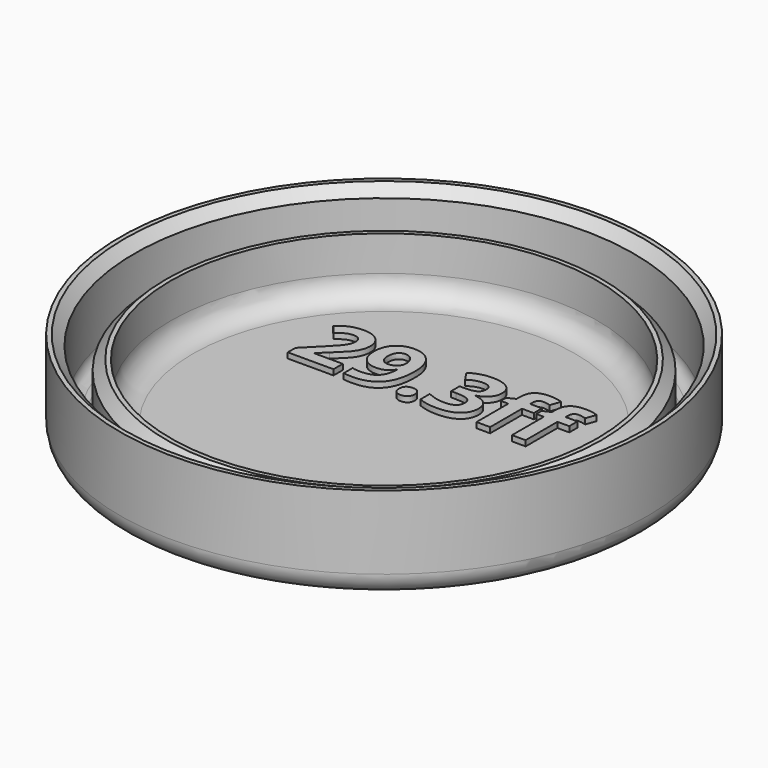
from build123d import *

# Parameters (mm, degrees)
F2_TEXT_SIZE = 8.3333333333
F3_DEPTH     = 0.5


# Not quite as in the source:
# - Text() gives the source's letters only with a copy of the font that has no kerning and outlines rounded to 1/6400 em; it was checked with that copy


with BuildPart() as f1:
    # F0 (on Front) → F1 (revolve)
    with BuildSketch(Plane.XZ):
        with BuildLine():
            Line((0, 1.5), (0, 0))
            Line((0, 0), (22, 0))
            ThreePointArc((22, 0), (23.4142135624, 0.5857864376), (24, 2))
            Line((24, 2), (24, 8.7))
            Line((24, 8.7), (23.6, 8.7))
            Line((23.6, 8.7), (22.7, 7.8))
            Line((22.7, 7.8), (22.7, 2.5))
            ThreePointArc((22.7, 2.5), (22.4071067812, 1.7928932188), (21.7, 1.5))
            Line((21.7, 1.5), (21.2, 1.5))
            ThreePointArc((21.2, 1.5), (20.8464466094, 1.6464466094), (20.7, 2))
            Line((20.7, 2), (20.7, 5.8))
            Line((20.7, 5.8), (19.8, 6.7))
            Line((19.8, 6.7), (19.4, 6.7))
            Line((19.4, 6.7), (19.4, 3.5))
            ThreePointArc((19.4, 3.5), (18.8142135624, 2.0857864376), (17.4, 1.5))
            Line((17.4, 1.5), (0, 1.5))
        make_face()
    revolve(axis=Axis((0, 0, 0.75), (0, 0, 1)))

    # F2 (on face) → F3 (join)
    with BuildSketch(Plane.XY.offset(1.5)):
        with Locations((-12.0071614583, 3.6423233468)):
            Text('29.3ff', F2_TEXT_SIZE, font='Open Sans', font_style=FontStyle.BOLD, text_align=(TextAlign.LEFT, TextAlign.BOTTOM))
    extrude(amount=F3_DEPTH)


solid = f1.part
